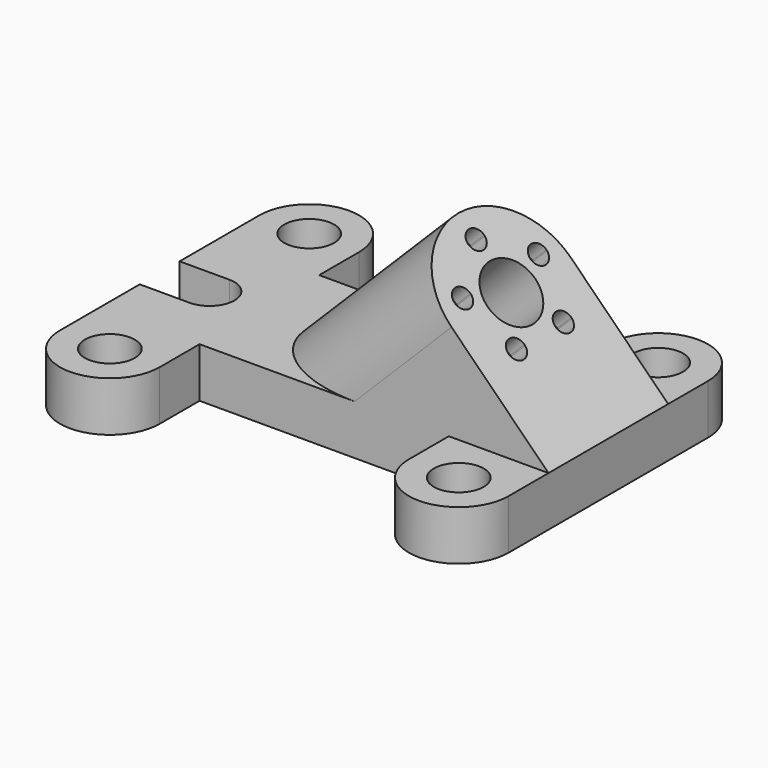
from build123d import *

# Parameters (mm, degrees)
F0_R             = 6.35
F1_DEPTH         = 12.7
F4_R             = 7.62
F6_DEPTH         = 5.08
F6_COPIES_COUNT  = 2
F6_COPIES_PITCH  = 14.929745
F6_COPIES1_COUNT = 2
F6_COPIES1_PITCH = 14.929745
F6_COPIES2_COUNT = 2
F6_COPIES2_PITCH = 24.156836
F6_COPIES3_COUNT = 2
F6_COPIES3_PITCH = 24.156836


# Not quite as in the source:
# - a pattern or mirror of a feature is missing from the dataset's text; its kind, count and spacing are read off the source's solid


with BuildPart() as f1:
    # F0 (on Top) → F1 (new body)
    with BuildSketch(Plane.XY):
        with BuildLine():
            Line((0, 31.75), (0, 6.35))
            Line((0, 6.35), (12.7, 6.35))
            ThreePointArc((12.7, 6.35), (17.1901280605, 4.4901280605), (19.05, 0))
            Line((19.05, 0), (114.3, 0))
            Line((114.3, 0), (114.3, 31.75))
            ThreePointArc((114.3, 31.75), (101.6, 44.45), (88.9, 31.75))
            Line((88.9, 31.75), (88.9, 19.05))
            Line((88.9, 19.05), (25.4, 19.05))
            Line((25.4, 19.05), (25.4, 31.75))
            ThreePointArc((25.4, 31.75), (12.7, 44.45), (0, 31.75))
        make_face()
        with Locations((12.7, 31.75)):
            Circle(F0_R, mode=Mode.SUBTRACT)
        with Locations((101.6, 31.75)):
            Circle(F0_R, mode=Mode.SUBTRACT)
    extrude(amount=F1_DEPTH)

    # F2: F1 across plane


with BuildPart() as f1_1:
    add(f1.part)
    add(f1.part.mirror(Plane.XZ))

    # F4 (on face) → F5 (join, up to the next surface of F1)
    with BuildSketch(Plane(origin=(63.5, 0, 63.5), x_dir=(0, 1, 0), z_dir=(0.7071067812, 0, 0.7071067812))):
        with BuildLine():
            Line((-19.05, -36.9170489686), (-19.05, -71.8420489686))
            Line((-19.05, -71.8420489686), (19.05, -71.8420489686))
            Line((19.05, -71.8420489686), (19.05, -36.9170489686))
            ThreePointArc((19.05, -36.9170489686), (0, -17.8670489686), (-19.05, -36.9170489686))
        make_face()
        with BuildLine():
            ThreePointArc((-2.5272680903, -24.4710489686), (-0.1271594487, -21.6802339429), (2.54, -24.2170489686))
            ThreePointArc((2.54, -24.2170489686), (2.5368150257, -24.3442084172), (2.5272680903, -24.4710489686))
            ThreePointArc((2.5272680903, -24.4710489686), (9.8332676346, -28.8798325582), (12.7, -36.9170489686))
            ThreePointArc((12.7, -36.9170489686), (-8.0372164104, -46.7503166031), (-2.5272680903, -24.4710489686))
        make_face(mode=Mode.SUBTRACT)
        with BuildLine():
            ThreePointArc((2.5272680903, -24.4710489686), (0, -26.7570489686), (-2.5272680903, -24.4710489686))
            ThreePointArc((-2.5272680903, -24.4710489686), (-8.0372164104, -46.7503166031), (12.7, -36.9170489686))
            ThreePointArc((12.7, -36.9170489686), (9.8332676346, -28.8798325582), (2.5272680903, -24.4710489686))
        make_face()
        with Locations((0, -36.9170489686)):
            Circle(F4_R, mode=Mode.SUBTRACT)
        with BuildLine():
            ThreePointArc((2.5272680903, -24.4710489686), (2.5368150257, -24.3442084172), (2.54, -24.2170489686))
            ThreePointArc((2.54, -24.2170489686), (-0.1271594487, -21.6802339429), (-2.5272680903, -24.4710489686))
            ThreePointArc((-2.5272680903, -24.4710489686), (0, -24.2170489686), (2.5272680903, -24.4710489686))
        make_face()
        with BuildLine():
            ThreePointArc((2.5272680903, -24.4710489686), (0, -24.2170489686), (-2.5272680903, -24.4710489686))
            ThreePointArc((-2.5272680903, -24.4710489686), (0, -26.7570489686), (2.5272680903, -24.4710489686))
        make_face()
    extrude(until=Until.NEXT, dir=(-0.7071067812, 0, -0.7071067812))

    # F4 (on face) → F6 (cut)
    with BuildSketch(Plane(origin=(63.5, 0, 63.5), x_dir=(0, 1, 0), z_dir=(0.7071067812, 0, 0.7071067812))):
        with BuildLine():
            ThreePointArc((2.5272680903, -24.4710489686), (2.5368150257, -24.3442084172), (2.54, -24.2170489686))
            ThreePointArc((2.54, -24.2170489686), (-0.1271594487, -21.6802339429), (-2.5272680903, -24.4710489686))
            ThreePointArc((-2.5272680903, -24.4710489686), (0, -24.2170489686), (2.5272680903, -24.4710489686))
        make_face()
        with BuildLine():
            ThreePointArc((2.5272680903, -24.4710489686), (0, -24.2170489686), (-2.5272680903, -24.4710489686))
            ThreePointArc((-2.5272680903, -24.4710489686), (0, -26.7570489686), (2.5272680903, -24.4710489686))
        make_face()
    f6 = extrude(amount=-F6_DEPTH, mode=Mode.SUBTRACT)

    # F6_copies: F6 ×2
    with Locations(*[Vector(0.4156269378, 0.8090169944, -0.4156269378) * (i * F6_COPIES_PITCH) for i in range(1, F6_COPIES_COUNT)]):
        add(f6, mode=Mode.SUBTRACT)

    # F6_copies1: F6 ×2
    with Locations(*[Vector(0.4156269378, -0.8090169944, -0.4156269378) * (i * F6_COPIES1_PITCH) for i in range(1, F6_COPIES1_COUNT)]):
        add(f6, mode=Mode.SUBTRACT)

    # F6_copies2: F6 ×2
    with Locations(*[Vector(0.672498512, -0.3090169944, -0.672498512) * (i * F6_COPIES2_PITCH) for i in range(1, F6_COPIES2_COUNT)]):
        add(f6, mode=Mode.SUBTRACT)

    # F6_copies3: F6 ×2
    with Locations(*[Vector(0.672498512, 0.3090169944, -0.672498512) * (i * F6_COPIES3_PITCH) for i in range(1, F6_COPIES3_COUNT)]):
        add(f6, mode=Mode.SUBTRACT)


solid = f1_1.part
